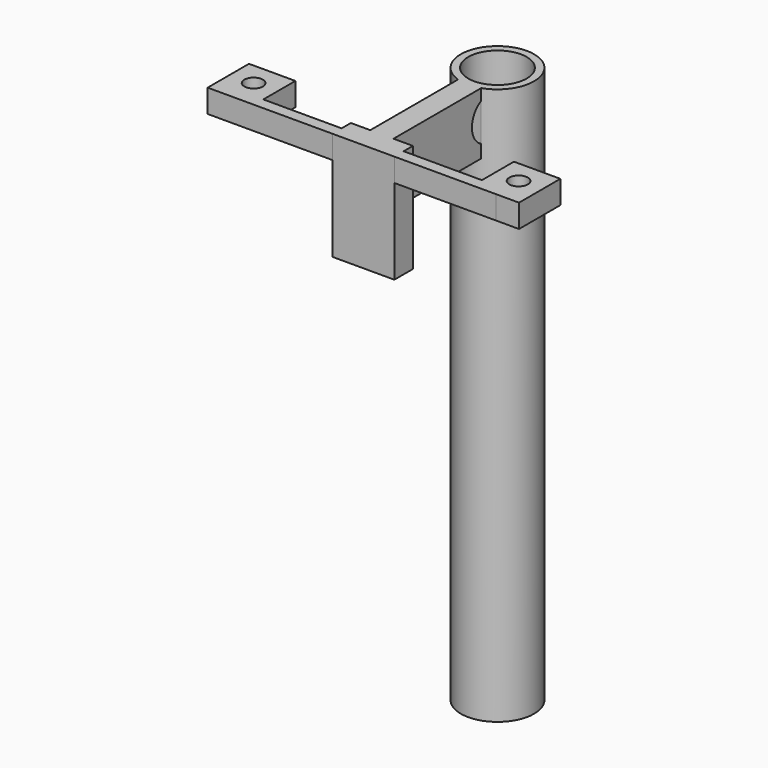
from build123d import *

# Parameters (mm, degrees)
F0_R     = 5.0165
F0_R_2   = 4.0005
F1_DEPTH = 76.2
F3_DEPTH = 8.4836
F5_DEPTH = 25.4
F7_DEPTH = 3.175
F8_W     = 8.4836
F8_H     = 3.175
F9_DEPTH = 6.35


# Not quite as in the source:
# - ends of sketch curves that miss each other by under 0.0002 mm in the source are joined


with BuildPart() as f1:
    # F0 (on Top) → F1 (new body)
    with BuildSketch(Plane.XY):
        Circle(F0_R)
        Circle(F0_R_2, mode=Mode.SUBTRACT)
    extrude(amount=F1_DEPTH)

    # F2 (on face) → F3 (join)
    with BuildSketch(Plane.XY.offset(76.2)):
        Polygon((-4.2418, -22.9430834), (0, -22.9430834), (4.2418, -22.9430834), (4.2418, -19.7680834), (1.5875, -19.7680834), (1.5875, -5.0165), (1.5875, -4.7586884748), (0, -4.7586884748), (-1.5875, -4.7586884748), (-1.5875, -19.7680834), (-4.2418, -19.7680834), align=None)
    extrude(amount=-F3_DEPTH)

    # F4 (on face) → F5 (cut)
    with BuildSketch(Plane.YZ.offset(1.5875)):
        with BuildLine():
            Line((-4.7586884748, 69.4789886475), (-4.7586884748, 74.6846720576))
            ThreePointArc((-4.7586884748, 74.6846720576), (-6.34993848, 72.0818303525), (-4.7586884748, 69.4789886475))
        make_face()
    extrude(amount=-F5_DEPTH, mode=Mode.SUBTRACT)

    # F6 (on face) → F7 (join)
    with BuildSketch(Plane.XY.offset(76.2)):
        Polygon((4.2418, -21.3555831969), (4.2418, -22.9430834), (18.1297326, -22.9430831969), (21.3047326, -22.9430831969), (21.3047326, -22.2236789969), (21.3047326, -15.8736789969), (14.9547326, -15.8736789969), (14.9547326, -21.3555831969), align=None)
        with BuildLine():
            ThreePointArc((18.1297326, -20.3186789969), (17.2317069879, -18.1506533848), (19.3997326, -19.0486789969))
            ThreePointArc((19.3997326, -19.0486789969), (19.0277582121, -19.946704609), (18.1297326, -20.3186789969))
        make_face(mode=Mode.SUBTRACT)
        Polygon((-4.2418, -22.9430831969), (0, -22.9430831969), (4.2418, -22.9430831969), (4.2418, -21.3555831969), (-4.2418, -21.3555831969), align=None)
        Polygon((-18.1297326, -22.9430831969), (-4.2418, -22.9430831969), (-4.2418, -21.3555831969), (-14.9547326, -21.3555831969), (-14.9547326, -15.8736789969), (-21.3047326, -15.8736789969), (-21.3047326, -22.2236789969), (-21.3047326, -22.9430831969), align=None)
        with BuildLine():
            ThreePointArc((-18.1297326, -20.3186789969), (-19.0277582121, -18.1506533848), (-16.8597326, -19.0486789969))
            ThreePointArc((-16.8597326, -19.0486789969), (-17.2317069879, -19.946704609), (-18.1297326, -20.3186789969))
        make_face(mode=Mode.SUBTRACT)
    extrude(amount=-F7_DEPTH)

    # F8 (on face) → F9 (join)
    with BuildSketch(Plane(origin=(0, 0, 67.7164), x_dir=(1, 0, 0), z_dir=(0, 0, -1))):
        with Locations((0, 21.3555834)):
            Rectangle(F8_W, F8_H)
    extrude(amount=F9_DEPTH)


solid = f1.part
